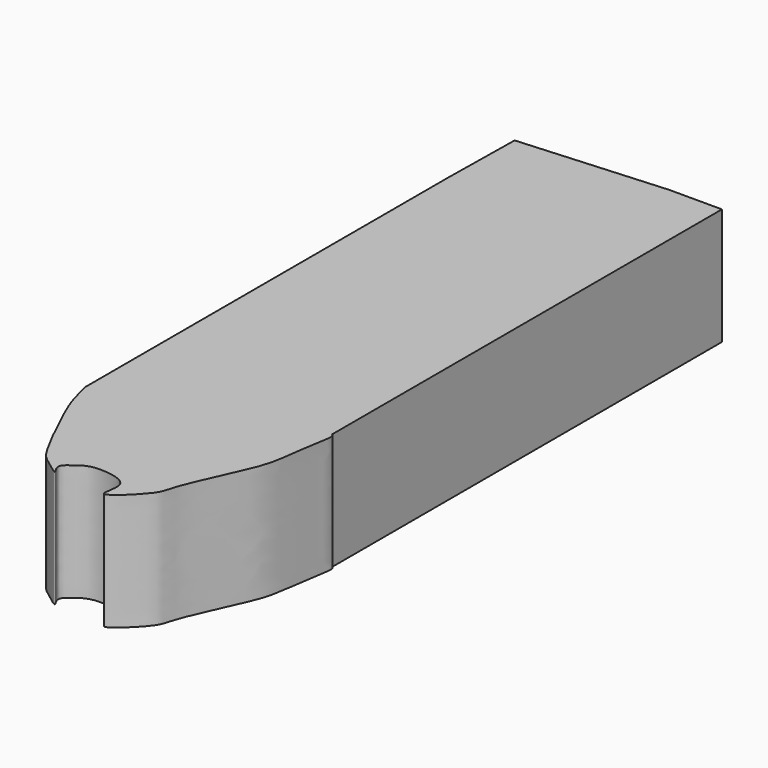
from build123d import *

# Parameters (mm, degrees)
F7_DEPTH  = 1123
F10_DEPTH = 233.1935763359


# Not quite as in the source:
# - the program builds the solid bodies; features that only make, move or delete a surface that nothing else refers to are left out


with BuildPart() as f7:
    # F6 (on offset) → F7 (new body)
    with BuildSketch(Plane.XZ.offset(-557.75)):
        Polygon((169.6261551561, -128.2491087914), (169.6261551561, 48.2507944107), (169.6261551561, 108.6985766888), (-169.2903935909, 108.6985766888), (-169.6261551561, 48.2507944107), (-169.6261551561, -128.2491087914), align=None)
    extrude(amount=F7_DEPTH)

    # F5 (on offset) → F10 (intersect)
    with BuildSketch(Plane.XY.offset(150.5)):
        with BuildLine():
            Line((-167.2138720751, 541.2015914917), (-179.2617440224, -240.8819943666))
            add(Edge.make_bspline(
                [(-179.2617440224, -240.8819943666), (-171.2785629658, -232.210792038), (-117.6374742605, -283.8445292108), (-17.1619143034, -305.5375031921), (70.5901704093, -300.5786903444), (148.8410396828, -237.3420253163), (159.273609519, -240.8819943666)],
                knots=[0, 0, 0, 0, 0.0527002892, 0.1215437511, 0.1860622975, 0.2501854479, 0.2501854479, 0.2501854479, 0.2501854479], degree=3))
            Line((159.273609519, -240.8819943666), (159.273609519, 563.7548832893))
            Line((159.273609519, 563.7548832893), (-167.2138720751, 541.2015914917))
        make_face()
        with BuildLine():
            add(Edge.make_bspline(
                [(-179.2617440224, -240.8819943666), (-171.2785629658, -232.210792038), (-117.6374742605, -283.8445292108), (-17.1619143034, -305.5375031921), (70.5901704093, -300.5786903444), (148.8410396828, -237.3420253163), (159.273609519, -240.8819943666)],
                knots=[0, 0, 0, 0, 0.0527002892, 0.1215437511, 0.1860622975, 0.2501854479, 0.2501854479, 0.2501854479, 0.2501854479], degree=3))
            add(Edge.make_bspline(
                [(159.273609519, -240.8819943666), (165.1715581046, -242.8832803184), (157.0677183853, -275.9768342439), (150.3335094214, -341.6566987697), (139.0113809757, -379.1436971228), (88.8013395888, -483.4680764953), (90.8664236555, -506.7081754017), (19.4131487824, -574.8080281458), (46.0341772666, -511.6650664223), (-1.2111921534, -500.9255535529), (-30.3744478627, -502.6420796901), (-48.3599921391, -516.2076109543), (-63.8333218342, -529.1135904742), (-44.4829025347, -551.8344123744), (-80.6953215397, -524.4251232165), (-97.5081138517, -511.1117853829), (-154.9211039076, -390.0627602909), (-163.2654628367, -360.8238205996), (-189.7149943602, -252.236146055), (-179.2617440224, -240.8819943666)],
                knots=[0.2501854479, 0.2501854479, 0.2501854479, 0.2501854479, 0.2864368271, 0.3410216598, 0.3854257032, 0.4538083426, 0.4913422386, 0.5435860815, 0.5804743356, 0.621504757, 0.6578574893, 0.6889370011, 0.7161093858, 0.7405245589, 0.7751164468, 0.8113243085, 0.8840177236, 0.930993759, 1, 1, 1, 1], degree=3))
        make_face()
    extrude(amount=-F10_DEPTH, mode=Mode.INTERSECT)


solid = f7.part
